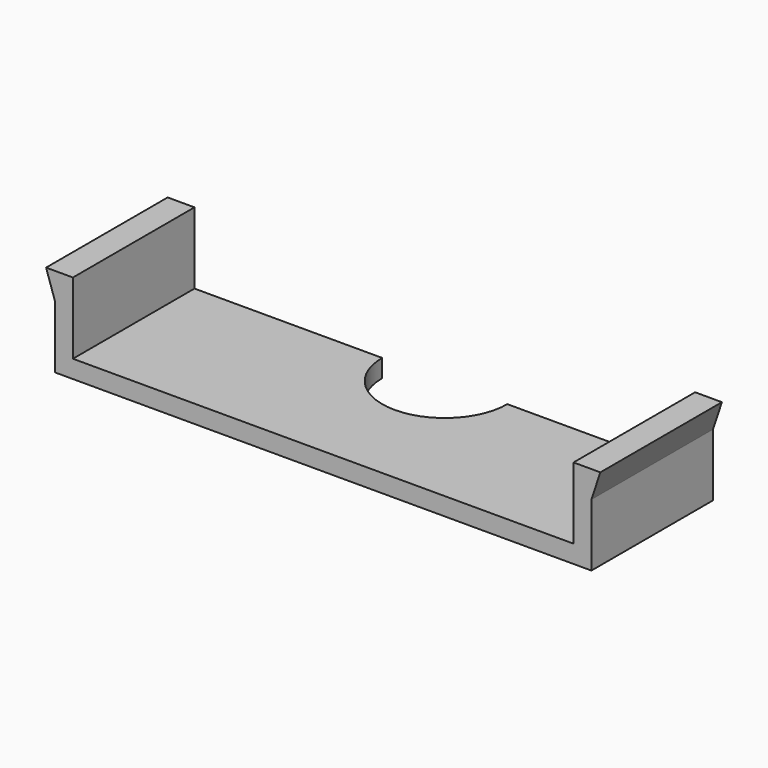
from build123d import *

# Parameters (mm, degrees)
F0_W     = 76.2
F0_H     = 21.59
F1_DEPTH = 2.54
F2_W     = 2.54
F2_H     = 21.59
F3_DEPTH = 10.16
F5_DEPTH = 25.4
F7_DEPTH = 21.59


# Not quite as in the source:
# - a feature names something its author has since deleted; it is built from what else it names


with BuildPart() as f1:
    # F0 (on Top) → F1 (new body)
    with BuildSketch(Plane.XY):
        with Locations((38.1, 10.795)):
            Rectangle(F0_W, F0_H)
    extrude(amount=F1_DEPTH)

    # F2 (on face) → F3 (join)
    with BuildSketch(Plane.XY.offset(2.54)):
        with Locations((1.27, 10.795)):
            Rectangle(F2_W, F2_H)
        with Locations((74.93, 10.795)):
            Rectangle(F2_W, F2_H)
    extrude(amount=F3_DEPTH)

    # F4 (on face) → F5 (cut)
    with BuildSketch(Plane.XY.offset(2.54)):
        with BuildLine():
            ThreePointArc((29.21, 21.59), (38.1, 12.7), (46.99, 21.59))
            Line((46.99, 21.59), (29.21, 21.59))
        make_face()
        with BuildLine():
            Line((29.21, 21.59), (46.99, 21.59))
            ThreePointArc((46.99, 21.59), (38.1, 30.48), (29.21, 21.59))
        make_face()
    extrude(amount=-F5_DEPTH, mode=Mode.SUBTRACT)

    # F6 (on face) → F7 (join, through all)
    with BuildSketch(Plane.XZ):
        Polygon((0, 8.89), (0, 12.7), (-1.27, 12.7), align=None)
        Polygon((76.2, 12.7), (76.2, 8.89), (77.47, 12.7), align=None)
    extrude(amount=-F7_DEPTH)


solid = f1.part
